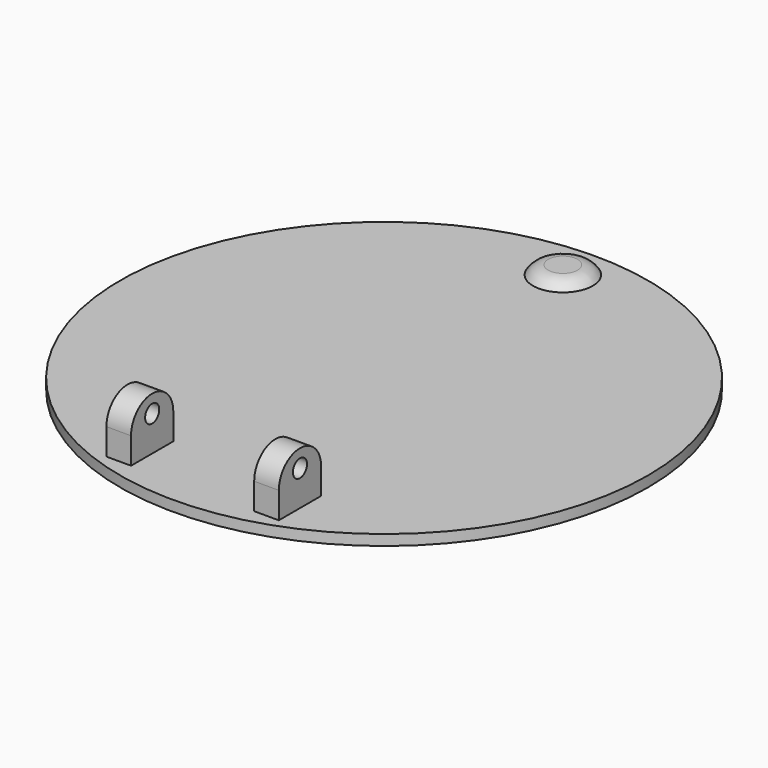
from build123d import *

# Parameters (mm, degrees)
F0_R     = 75
F0_W     = 7
F0_H     = 15
F1_DEPTH = 3
F2_DEPTH = 15
F3_R     = 2.5
F4_DEPTH = 99.4959988723
F5_R     = 8.5
F6_DEPTH = 2.5
F6_TAPER = 10


# Not quite as in the source:
# - a fillet or chamfer that OpenCascade refuses, or shapes differently, is made with other operations: its cross-section is extruded or revolved along the edge and cut away or added


with BuildPart() as f1:
    # F0 (on Top) → F1 (new body)
    with BuildSketch(Plane.XY):
        Circle(F0_R)
        with Locations((-20.9949988723, -60.5)):
            Rectangle(F0_W, F0_H, mode=Mode.SUBTRACT)
        with Locations((20.9949988723, -60.5)):
            Rectangle(F0_W, F0_H, mode=Mode.SUBTRACT)
        with Locations((-20.9949988723, -60.5)):
            Rectangle(F0_W, F0_H)
        with Locations((20.9949988723, -60.5)):
            Rectangle(F0_W, F0_H)
    extrude(amount=-F1_DEPTH)

    # F0 (on Top) → F2 (join)
    with BuildSketch(Plane.XY):
        with Locations((20.9949988723, -60.5)):
            Rectangle(F0_W, F0_H)
        with Locations((-20.9949988723, -60.5)):
            Rectangle(F0_W, F0_H)
    extrude(amount=F2_DEPTH)

    # F3 (on face) → F4 (cut, through all)
    with BuildSketch(Plane.YZ.offset(24.4949988723)):
        with BuildLine():
            ThreePointArc((-68, 7.5), (-65.8033008589, 12.8033008589), (-60.5, 15))
            Line((-60.5, 15), (-68, 15))
            Line((-68, 15), (-68, 7.5))
        make_face()
        with BuildLine():
            ThreePointArc((-60.5, 15), (-55.1966991411, 12.8033008589), (-53, 7.5))
            Line((-53, 7.5), (-53, 15))
            Line((-53, 15), (-60.5, 15))
        make_face()
        with Locations((-60.5, 10)):
            Circle(F3_R)
    extrude(amount=-F4_DEPTH, mode=Mode.SUBTRACT)

    # F5 (on face) → F6 (join)
    with BuildSketch(Plane.XY):
        with Locations((0, 63.5)):
            Circle(F5_R)
    extrude(amount=F6_DEPTH, taper=F6_TAPER)

    # F7: fillet of radius 5 on 1 edges, made by hand

    # F7_s1 → F7_t2 (revolve, cut)
    with BuildSketch(Plane.XZ.offset(-63.5)):
        with BuildLine():
            ThreePointArc((8.5, 0), (6.6698729811, 1.8301270189), (4.1698729811, 2.5))
            Line((4.1698729811, 2.5), (8.0591825482, 2.5))
            Line((8.0591825482, 2.5), (8.5, 0))
        make_face()
    revolve(axis=Axis((0, 63.5, 2.5), (0, 0, -1)), mode=Mode.SUBTRACT)


solid = f1.part
